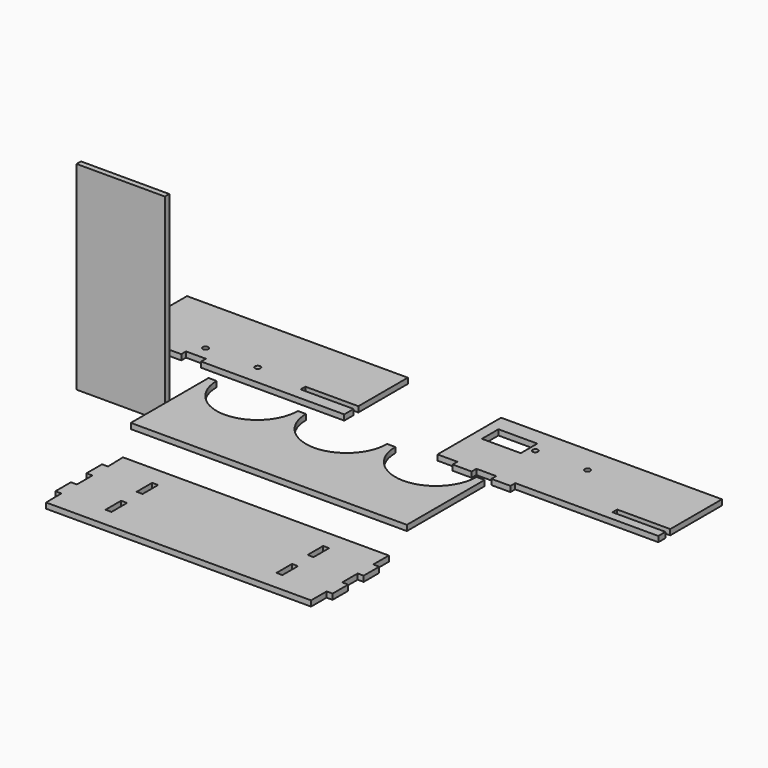
from build123d import *

# Parameters (mm, degrees)
F1_DEPTH = 3.175
F2_R     = 1.5875
F3_DEPTH = 3.175
F4_W     = 3.429
F4_H     = 11.176
F5_DEPTH = 3.175
F6_W     = 22.352
F6_H     = 11.90625
F6_R     = 1.5875
F7_DEPTH = 3.175
F8_W     = 50.8
F8_H     = 114.3
F9_DEPTH = 3.175


# Not quite as in the source:
# - a length typed as a fraction of an inch, garbled in the dataset ("3 / 203.2 mm" for 3/8 in), is restored


with BuildPart() as f1:
    # F0 (on Top) → F1 (new body)
    with BuildSketch(Plane.XY):
        with BuildLine():
            Line((-72.0875338231, 25.7993119954), (-76.7230338231, 25.7993119954))
            Line((-76.7230338231, 25.7993119954), (-76.7230338231, -30.0806880046))
            Line((-76.7230338231, -30.0806880046), (82.0269661769, -30.0806880046))
            Line((82.0269661769, -30.0806880046), (82.0269661769, 25.7993119954))
            Line((82.0269661769, 25.7993119954), (77.3914661769, 25.7993119954))
            ThreePointArc((77.3914661769, 25.7993119954), (54.0234661769, 2.4313119954), (30.6554661769, 25.7993119954))
            Line((30.6554661769, 25.7993119954), (26.0199661769, 25.7993119954))
            ThreePointArc((26.0199661769, 25.7993119954), (2.6519661769, 2.4313119954), (-20.7160338231, 25.7993119954))
            Line((-20.7160338231, 25.7993119954), (-25.3515338231, 25.7993119954))
            ThreePointArc((-25.3515338231, 25.7993119954), (-48.7195338231, 2.4313119954), (-72.0875338231, 25.7993119954))
        make_face()
    extrude(amount=F1_DEPTH)


with BuildPart() as f3:
    # F2 (on Top) → F3 (new body)
    with BuildSketch(Plane.XY):
        Polygon((-7.0445054214, 81.9526092303), (-134.0445054214, 81.9526092303), (-134.0445054214, 36.2326092303), (-123.1225054214, 36.2326092303), (-123.1225054214, 39.6616092303), (-111.6925054214, 39.6616092303), (-111.6925054214, 36.2326092303), (-100.7705054214, 36.2326092303), (-100.7705054214, 39.6616092303), (-89.3405054214, 39.6616092303), (-89.3405054214, 36.2326092303), (-78.4185054214, 36.2326092303), (-66.9885054214, 36.2326092303), (-7.0445054214, 36.2326092303), (-7.0445054214, 42.9636092303), (-37.5245054214, 42.9636092303), (-37.5245054214, 46.3926092303), (-7.0445054214, 46.3926092303), align=None)
        with Locations((-95.9445054214, 47.6880092303)):
            Circle(F2_R, mode=Mode.SUBTRACT)
        with Locations((-65.9445054214, 47.6880092303)):
            Circle(F2_R, mode=Mode.SUBTRACT)
    extrude(amount=F3_DEPTH)


with BuildPart() as f5:
    # F4 (on Top) → F5 (new body)
    with BuildSketch(Plane.XY):
        Polygon((94.330517361, -58.446758062), (-58.5715263949, -58.446758062), (-58.2169860113, -69.6171330385), (-61.6459860113, -69.6171330385), (-61.6459860113, -80.7931330385), (-58.2169860113, -80.7931330385), (-58.2169860113, -91.9691330385), (-61.6459860113, -91.9691330385), (-61.6459860113, -103.1517314958), (-58.2169860113, -103.1517314958), (-58.069482639, -114.326758062), (94.330517361, -114.326758062), (94.330517361, -103.150758062), (97.759517361, -103.150758062), (97.759517361, -91.974758062), (94.330517361, -91.974758062), (94.330517361, -80.798758062), (97.759517361, -80.798758062), (97.759517361, -69.622758062), (94.330517361, -69.622758062), align=None)
        with Locations((-31.1024860113, -97.562758062)):
            Rectangle(F4_W, F4_H, mode=Mode.SUBTRACT)
        with Locations((67.216017361, -97.562758062)):
            Rectangle(F4_W, F4_H, mode=Mode.SUBTRACT)
        with Locations((-31.1024860113, -75.210758062)):
            Rectangle(F4_W, F4_H, mode=Mode.SUBTRACT)
        with Locations((67.216017361, -75.210758062)):
            Rectangle(F4_W, F4_H, mode=Mode.SUBTRACT)
    extrude(amount=F5_DEPTH)


with BuildPart() as f7:
    # F6 (on Top) → F7 (new body)
    with BuildSketch(Plane.XY):
        Polygon((176.9865440756, 77.7137125557), (49.9865440756, 77.7137125557), (49.9865440756, 31.9937125557), (61.4165440756, 31.9937125557), (61.4165440756, 28.5647125557), (72.3385440756, 28.5647125557), (72.3385440756, 31.9937125557), (83.7685440756, 31.9937125557), (83.7685440756, 28.5647125557), (94.6905440756, 28.5647125557), (94.6905440756, 31.9937125557), (176.9865440756, 31.9937125557), (176.9865440756, 37.1372125557), (146.5065440756, 37.1372125557), (146.5065440756, 40.5662125557), (176.9865440756, 40.5662125557), align=None)
        with Locations((67.2585440756, 62.2355875557)):
            Rectangle(F6_W, F6_H, mode=Mode.SUBTRACT)
        with Locations((82.0845440756, 62.2324125557)):
            Circle(F6_R, mode=Mode.SUBTRACT)
        with Locations((112.0845440756, 62.2324125557)):
            Circle(F6_R, mode=Mode.SUBTRACT)
    extrude(amount=F7_DEPTH)


with BuildPart() as f9:
    # F8 (on Front) → F9 (new body)
    with BuildSketch(Plane.XZ):
        with Locations((-104.0762934036, 49.0330420434)):
            Rectangle(F8_W, F8_H)
    extrude(amount=F9_DEPTH)


solid = Compound([f1.part, f3.part, f5.part, f7.part, f9.part])
